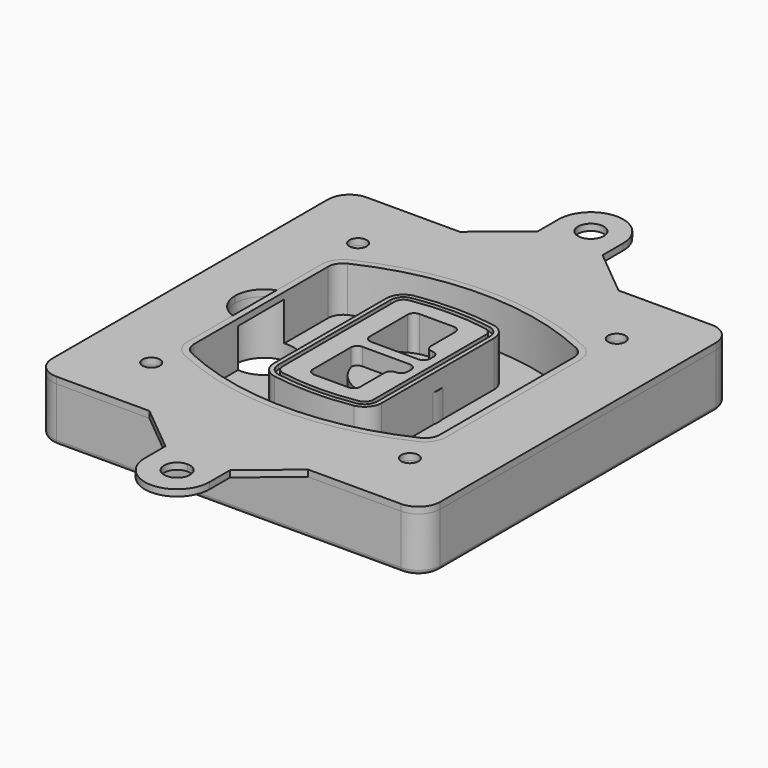
from build123d import *

# Parameters (mm, degrees)
F0_R      = 4
F1_DEPTH  = 25
F2_DEPTH  = 3
F3_DEPTH  = 18
F5_DEPTH  = 21
F6_DEPTH  = 2
F8_DEPTH  = 20
F9_DEPTH  = 16
F10_DEPTH = 25
F7_R      = 6
F7_R_2    = 4
F11_DEPTH = 6
F13_DEPTH = 9
F14_R     = 2
F15_R     = 4
F16_DEPTH = 3


# Not quite as in the source:
# - a feature names something its author has since deleted; it is built from what else it names


with BuildPart() as f1:
    # F0 (on Top) → F1 (new body)
    with BuildSketch(Plane.XY):
        with BuildLine():
            ThreePointArc((-90, -80), (-87.0710678119, -87.0710678119), (-80, -90))
            Line((-80, -90), (80, -90))
            ThreePointArc((80, -90), (87.0710678119, -87.0710678119), (90, -80))
            Line((90, -80), (90, 80))
            ThreePointArc((90, 80), (87.0710678119, 87.0710678119), (80, 90))
            Line((80, 90), (-80, 90))
            ThreePointArc((-80, 90), (-87.0710678119, 87.0710678119), (-90, 80))
            Line((-90, 80), (-90, -80))
        make_face()
        with Locations((-60, -60)):
            Circle(F0_R, mode=Mode.SUBTRACT)
        with Locations((60, -60)):
            Circle(F0_R, mode=Mode.SUBTRACT)
        with BuildLine():
            ThreePointArc((-64, 38.8308515907), (-61.8195654598, 46.3340424013), (-55.9574468085, 51.5000594398))
            ThreePointArc((-55.9574468085, 51.5000594398), (0, 64), (55.9574468085, 51.5000594398))
            ThreePointArc((55.9574468085, 51.5000594398), (61.8195654598, 46.3340424013), (64, 38.8308515907))
            Line((64, 38.8308515907), (64, -38.8308515907))
            ThreePointArc((64, -38.8308515907), (61.8195654598, -46.3340424013), (55.9574468085, -51.5000594398))
            ThreePointArc((55.9574468085, -51.5000594398), (0, -64), (-55.9574468085, -51.5000594398))
            ThreePointArc((-55.9574468085, -51.5000594398), (-61.8195654598, -46.3340424013), (-64, -38.8308515907))
            Line((-64, -38.8308515907), (-64, 38.8308515907))
        make_face(mode=Mode.SUBTRACT)
        with Locations((-60, 60)):
            Circle(F0_R, mode=Mode.SUBTRACT)
        with Locations((60, 60)):
            Circle(F0_R, mode=Mode.SUBTRACT)
        with BuildLine():
            ThreePointArc((55.9574468085, 51.5000594398), (0, 64), (-55.9574468085, 51.5000594398))
            ThreePointArc((-55.9574468085, 51.5000594398), (-61.8195654598, 46.3340424013), (-64, 38.8308515907))
            Line((-64, 38.8308515907), (-64, -38.8308515907))
            ThreePointArc((-64, -38.8308515907), (-61.8195654598, -46.3340424013), (-55.9574468085, -51.5000594398))
            ThreePointArc((-55.9574468085, -51.5000594398), (0, -64), (55.9574468085, -51.5000594398))
            ThreePointArc((55.9574468085, -51.5000594398), (61.8195654598, -46.3340424013), (64, -38.8308515907))
            Line((64, -38.8308515907), (64, 38.8308515907))
            ThreePointArc((64, 38.8308515907), (61.8195654598, 46.3340424013), (55.9574468085, 51.5000594398))
        make_face()
        with BuildLine():
            Line((-60, -38.8308515907), (-60, 38.8308515907))
            ThreePointArc((-60, 38.8308515907), (-58.442546757, 44.1902735983), (-54.2553191489, 47.8802857686))
            ThreePointArc((-54.2553191489, 47.8802857686), (0, 60), (54.2553191489, 47.8802857686))
            ThreePointArc((54.2553191489, 47.8802857686), (58.442546757, 44.1902735983), (60, 38.8308515907))
            Line((60, 38.8308515907), (60, -38.8308515907))
            ThreePointArc((60, -38.8308515907), (58.442546757, -44.1902735983), (54.2553191489, -47.8802857686))
            ThreePointArc((54.2553191489, -47.8802857686), (0, -60), (-54.2553191489, -47.8802857686))
            ThreePointArc((-54.2553191489, -47.8802857686), (-58.442546757, -44.1902735983), (-60, -38.8308515907))
        make_face(mode=Mode.SUBTRACT)
        with BuildLine():
            ThreePointArc((-54.2553191489, 47.8802857686), (-58.442546757, 44.1902735983), (-60, 38.8308515907))
            Line((-60, 38.8308515907), (-60, -38.8308515907))
            ThreePointArc((-60, -38.8308515907), (-58.442546757, -44.1902735983), (-54.2553191489, -47.8802857686))
            ThreePointArc((-54.2553191489, -47.8802857686), (0, -60), (54.2553191489, -47.8802857686))
            ThreePointArc((54.2553191489, -47.8802857686), (58.442546757, -44.1902735983), (60, -38.8308515907))
            Line((60, -38.8308515907), (60, 38.8308515907))
            ThreePointArc((60, 38.8308515907), (58.442546757, 44.1902735983), (54.2553191489, 47.8802857686))
            ThreePointArc((54.2553191489, 47.8802857686), (0, 60), (-54.2553191489, 47.8802857686))
        make_face()
        with BuildLine():
            ThreePointArc((52.9787234043, 45.1654555152), (55.9097827299, 42.582446996), (57, 38.8308515907))
            Line((57, 38.8308515907), (57, -38.8308515907))
            ThreePointArc((57, -38.8308515907), (55.9097827299, -42.582446996), (52.9787234043, -45.1654555152))
            ThreePointArc((52.9787234043, -45.1654555152), (0, -57), (-52.9787234043, -45.1654555152))
            ThreePointArc((-52.9787234043, -45.1654555152), (-55.9097827299, -42.582446996), (-57, -38.8308515907))
            Line((-57, -38.8308515907), (-57, 38.8308515907))
            ThreePointArc((-57, 38.8308515907), (-55.9097827299, 42.582446996), (-52.9787234043, 45.1654555152))
            ThreePointArc((-52.9787234043, 45.1654555152), (0, 57), (52.9787234043, 45.1654555152))
        make_face(mode=Mode.SUBTRACT)
        with BuildLine():
            Line((57, -38.8308515907), (57, 38.8308515907))
            ThreePointArc((57, 38.8308515907), (55.9097827299, 42.582446996), (52.9787234043, 45.1654555152))
            ThreePointArc((52.9787234043, 45.1654555152), (0, 57), (-52.9787234043, 45.1654555152))
            ThreePointArc((-52.9787234043, 45.1654555152), (-55.9097827299, 42.582446996), (-57, 38.8308515907))
            Line((-57, 38.8308515907), (-57, -38.8308515907))
            ThreePointArc((-57, -38.8308515907), (-55.9097827299, -42.582446996), (-52.9787234043, -45.1654555152))
            ThreePointArc((-52.9787234043, -45.1654555152), (0, -57), (52.9787234043, -45.1654555152))
            ThreePointArc((52.9787234043, -45.1654555152), (55.9097827299, -42.582446996), (57, -38.8308515907))
        make_face()
    extrude(amount=-F1_DEPTH)

    # F0 (on Top) → F2 (join)
    with BuildSketch(Plane.XY):
        with BuildLine():
            ThreePointArc((-54.2553191489, 47.8802857686), (-58.442546757, 44.1902735983), (-60, 38.8308515907))
            Line((-60, 38.8308515907), (-60, -38.8308515907))
            ThreePointArc((-60, -38.8308515907), (-58.442546757, -44.1902735983), (-54.2553191489, -47.8802857686))
            ThreePointArc((-54.2553191489, -47.8802857686), (0, -60), (54.2553191489, -47.8802857686))
            ThreePointArc((54.2553191489, -47.8802857686), (58.442546757, -44.1902735983), (60, -38.8308515907))
            Line((60, -38.8308515907), (60, 38.8308515907))
            ThreePointArc((60, 38.8308515907), (58.442546757, 44.1902735983), (54.2553191489, 47.8802857686))
            ThreePointArc((54.2553191489, 47.8802857686), (0, 60), (-54.2553191489, 47.8802857686))
        make_face()
        with BuildLine():
            ThreePointArc((52.9787234043, 45.1654555152), (55.9097827299, 42.582446996), (57, 38.8308515907))
            Line((57, 38.8308515907), (57, -38.8308515907))
            ThreePointArc((57, -38.8308515907), (55.9097827299, -42.582446996), (52.9787234043, -45.1654555152))
            ThreePointArc((52.9787234043, -45.1654555152), (0, -57), (-52.9787234043, -45.1654555152))
            ThreePointArc((-52.9787234043, -45.1654555152), (-55.9097827299, -42.582446996), (-57, -38.8308515907))
            Line((-57, -38.8308515907), (-57, 38.8308515907))
            ThreePointArc((-57, 38.8308515907), (-55.9097827299, 42.582446996), (-52.9787234043, 45.1654555152))
            ThreePointArc((-52.9787234043, 45.1654555152), (0, 57), (52.9787234043, 45.1654555152))
        make_face(mode=Mode.SUBTRACT)
    extrude(amount=F2_DEPTH)

    # F0 (on Top) → F3 (cut)
    with BuildSketch(Plane.XY):
        with BuildLine():
            Line((57, -38.8308515907), (57, 38.8308515907))
            ThreePointArc((57, 38.8308515907), (55.9097827299, 42.582446996), (52.9787234043, 45.1654555152))
            ThreePointArc((52.9787234043, 45.1654555152), (0, 57), (-52.9787234043, 45.1654555152))
            ThreePointArc((-52.9787234043, 45.1654555152), (-55.9097827299, 42.582446996), (-57, 38.8308515907))
            Line((-57, 38.8308515907), (-57, -38.8308515907))
            ThreePointArc((-57, -38.8308515907), (-55.9097827299, -42.582446996), (-52.9787234043, -45.1654555152))
            ThreePointArc((-52.9787234043, -45.1654555152), (0, -57), (52.9787234043, -45.1654555152))
            ThreePointArc((52.9787234043, -45.1654555152), (55.9097827299, -42.582446996), (57, -38.8308515907))
        make_face()
    extrude(amount=-F3_DEPTH, mode=Mode.SUBTRACT)

    # F4 (on face) → F5 (join, through all)
    with BuildSketch(Plane.XY.offset(3)):
        with BuildLine():
            ThreePointArc((-25, -32.5662280692), (-23.1122504785, -37.7276614059), (-18.3399014778, -40.4532214146))
            ThreePointArc((-18.3399014778, -40.4532214146), (0, -42), (18.3399014778, -40.4532214146))
            ThreePointArc((18.3399014778, -40.4532214146), (23.1122504785, -37.7276614059), (25, -32.5662280692))
            Line((25, -32.5662280692), (25, 32.5662280692))
            ThreePointArc((25, 32.5662280692), (23.1122504785, 37.7276614059), (18.3399014778, 40.4532214146))
            ThreePointArc((18.3399014778, 40.4532214146), (0, 42), (-18.3399014778, 40.4532214146))
            ThreePointArc((-18.3399014778, 40.4532214146), (-23.1122504785, 37.7276614059), (-25, 32.5662280692))
            Line((-25, 32.5662280692), (-25, -32.5662280692))
        make_face()
        with BuildLine():
            ThreePointArc((18.0049261084, 38.4814730782), (21.5841878588, 36.4373030717), (23, 32.5662280692))
            Line((23, 32.5662280692), (23, -32.5662280692))
            ThreePointArc((23, -32.5662280692), (21.5841878588, -36.4373030717), (18.0049261084, -38.4814730782))
            ThreePointArc((18.0049261084, -38.4814730782), (0, -40), (-18.0049261084, -38.4814730782))
            ThreePointArc((-18.0049261084, -38.4814730782), (-21.5841878588, -36.4373030717), (-23, -32.5662280692))
            Line((-23, -32.5662280692), (-23, 32.5662280692))
            ThreePointArc((-23, 32.5662280692), (-21.5841878588, 36.4373030717), (-18.0049261084, 38.4814730782))
            ThreePointArc((-18.0049261084, 38.4814730782), (0, 40), (18.0049261084, 38.4814730782))
        make_face(mode=Mode.SUBTRACT)
        with BuildLine():
            Line((23, -32.5662280692), (23, 32.5662280692))
            ThreePointArc((23, 32.5662280692), (21.5841878588, 36.4373030717), (18.0049261084, 38.4814730782))
            ThreePointArc((18.0049261084, 38.4814730782), (0, 40), (-18.0049261084, 38.4814730782))
            ThreePointArc((-18.0049261084, 38.4814730782), (-21.5841878588, 36.4373030717), (-23, 32.5662280692))
            Line((-23, 32.5662280692), (-23, -32.5662280692))
            ThreePointArc((-23, -32.5662280692), (-21.5841878588, -36.4373030717), (-18.0049261084, -38.4814730782))
            ThreePointArc((-18.0049261084, -38.4814730782), (0, -40), (18.0049261084, -38.4814730782))
            ThreePointArc((18.0049261084, -38.4814730782), (21.5841878588, -36.4373030717), (23, -32.5662280692))
        make_face()
        with BuildLine():
            ThreePointArc((17.6699507389, 36.5097247419), (20.0561252392, 35.1469447375), (21, 32.5662280692))
            Line((21, 32.5662280692), (21, -32.5662280692))
            ThreePointArc((21, -32.5662280692), (20.0561252392, -35.1469447375), (17.6699507389, -36.5097247419))
            ThreePointArc((17.6699507389, -36.5097247419), (0, -38), (-17.6699507389, -36.5097247419))
            ThreePointArc((-17.6699507389, -36.5097247419), (-20.0561252392, -35.1469447375), (-21, -32.5662280692))
            Line((-21, -32.5662280692), (-21, 32.5662280692))
            ThreePointArc((-21, 32.5662280692), (-20.0561252392, 35.1469447375), (-17.6699507389, 36.5097247419))
            ThreePointArc((-17.6699507389, 36.5097247419), (0, 38), (17.6699507389, 36.5097247419))
        make_face(mode=Mode.SUBTRACT)
        with BuildLine():
            Line((21, -32.5662280692), (21, 32.5662280692))
            ThreePointArc((21, 32.5662280692), (20.0561252392, 35.1469447375), (17.6699507389, 36.5097247419))
            ThreePointArc((17.6699507389, 36.5097247419), (0, 38), (-17.6699507389, 36.5097247419))
            ThreePointArc((-17.6699507389, 36.5097247419), (-20.0561252392, 35.1469447375), (-21, 32.5662280692))
            Line((-21, 32.5662280692), (-21, -32.5662280692))
            ThreePointArc((-21, -32.5662280692), (-20.0561252392, -35.1469447375), (-17.6699507389, -36.5097247419))
            ThreePointArc((-17.6699507389, -36.5097247419), (0, -38), (17.6699507389, -36.5097247419))
            ThreePointArc((17.6699507389, -36.5097247419), (20.0561252392, -35.1469447375), (21, -32.5662280692))
        make_face()
        with BuildLine():
            Line((-8, -2.5), (14, -2.5))
            ThreePointArc((14, -2.5), (16.1213203436, -3.3786796564), (17, -5.5))
            Line((17, -5.5), (17, -7.5))
            ThreePointArc((17, -7.5), (16.1213203436, -9.6213203436), (14, -10.5))
            ThreePointArc((14, -10.5), (11.8786796564, -11.3786796564), (11, -13.5))
            Line((11, -13.5), (11, -27.5))
            ThreePointArc((11, -27.5), (10.1213203436, -29.6213203436), (8, -30.5))
            Line((8, -30.5), (-8, -30.5))
            ThreePointArc((-8, -30.5), (-10.1213203436, -29.6213203436), (-11, -27.5))
            Line((-11, -27.5), (-11, -5.5))
            ThreePointArc((-11, -5.5), (-10.1213203436, -3.3786796564), (-8, -2.5))
        make_face(mode=Mode.SUBTRACT)
        with BuildLine():
            ThreePointArc((-8, 2.5), (-10.1213203436, 3.3786796564), (-11, 5.5))
            Line((-11, 5.5), (-11, 27.5))
            ThreePointArc((-11, 27.5), (-10.1213203436, 29.6213203436), (-8, 30.5))
            Line((-8, 30.5), (8, 30.5))
            ThreePointArc((8, 30.5), (10.1213203436, 29.6213203436), (11, 27.5))
            Line((11, 27.5), (11, 13.5))
            ThreePointArc((11, 13.5), (11.8786796564, 11.3786796564), (14, 10.5))
            ThreePointArc((14, 10.5), (16.1213203436, 9.6213203436), (17, 7.5))
            Line((17, 7.5), (17, 5.5))
            ThreePointArc((17, 5.5), (16.1213203436, 3.3786796564), (14, 2.5))
            Line((14, 2.5), (-8, 2.5))
        make_face(mode=Mode.SUBTRACT)
    extrude(amount=-F5_DEPTH)

    # F4 (on face) → F6 (cut)
    with BuildSketch(Plane.XY.offset(3)):
        with BuildLine():
            Line((23, -32.5662280692), (23, 32.5662280692))
            ThreePointArc((23, 32.5662280692), (21.5841878588, 36.4373030717), (18.0049261084, 38.4814730782))
            ThreePointArc((18.0049261084, 38.4814730782), (0, 40), (-18.0049261084, 38.4814730782))
            ThreePointArc((-18.0049261084, 38.4814730782), (-21.5841878588, 36.4373030717), (-23, 32.5662280692))
            Line((-23, 32.5662280692), (-23, -32.5662280692))
            ThreePointArc((-23, -32.5662280692), (-21.5841878588, -36.4373030717), (-18.0049261084, -38.4814730782))
            ThreePointArc((-18.0049261084, -38.4814730782), (0, -40), (18.0049261084, -38.4814730782))
            ThreePointArc((18.0049261084, -38.4814730782), (21.5841878588, -36.4373030717), (23, -32.5662280692))
        make_face()
        with BuildLine():
            ThreePointArc((17.6699507389, 36.5097247419), (20.0561252392, 35.1469447375), (21, 32.5662280692))
            Line((21, 32.5662280692), (21, -32.5662280692))
            ThreePointArc((21, -32.5662280692), (20.0561252392, -35.1469447375), (17.6699507389, -36.5097247419))
            ThreePointArc((17.6699507389, -36.5097247419), (0, -38), (-17.6699507389, -36.5097247419))
            ThreePointArc((-17.6699507389, -36.5097247419), (-20.0561252392, -35.1469447375), (-21, -32.5662280692))
            Line((-21, -32.5662280692), (-21, 32.5662280692))
            ThreePointArc((-21, 32.5662280692), (-20.0561252392, 35.1469447375), (-17.6699507389, 36.5097247419))
            ThreePointArc((-17.6699507389, 36.5097247419), (0, 38), (17.6699507389, 36.5097247419))
        make_face(mode=Mode.SUBTRACT)
    extrude(amount=-F6_DEPTH, mode=Mode.SUBTRACT)

    # F7 (on face) → F8 (join)
    with BuildSketch(Plane(origin=(0, 0, -25), x_dir=(1, 0, 0), z_dir=(0, 0, -1))):
        with BuildLine():
            ThreePointArc((-6.71157564, 0), (6.7567035675, 13.4682792075), (20.224982775, 0))
            Line((20.224982775, 0), (25.224982775, 0))
            ThreePointArc((25.224982775, 0), (6.7567035675, 18.4682792075), (-11.71157564, 0))
            Line((-11.71157564, 0), (-6.71157564, 0))
        make_face()
        with BuildLine():
            Line((-6.71157564, 0), (20.224982775, 0))
            ThreePointArc((20.224982775, 0), (6.7567035675, 13.4682792075), (-6.71157564, 0))
        make_face()
        with BuildLine():
            ThreePointArc((-6.71157564, 0), (6.7567035675, -13.4682792075), (20.224982775, 0))
            Line((20.224982775, 0), (-6.71157564, 0))
        make_face()
        with BuildLine():
            Line((25.224982775, 0), (20.224982775, 0))
            ThreePointArc((20.224982775, 0), (6.7567035675, -13.4682792075), (-6.71157564, 0))
            Line((-6.71157564, 0), (-11.71157564, 0))
            ThreePointArc((-11.71157564, 0), (6.7567035675, -18.4682792075), (25.224982775, 0))
        make_face()
    extrude(amount=-F8_DEPTH)

    # F7 (on face) → F9 (cut)
    with BuildSketch(Plane(origin=(0, 0, -25), x_dir=(1, 0, 0), z_dir=(0, 0, -1))):
        with BuildLine():
            Line((-6.71157564, 0), (20.224982775, 0))
            ThreePointArc((20.224982775, 0), (6.7567035675, 13.4682792075), (-6.71157564, 0))
        make_face()
        with BuildLine():
            ThreePointArc((-6.71157564, 0), (6.7567035675, -13.4682792075), (20.224982775, 0))
            Line((20.224982775, 0), (-6.71157564, 0))
        make_face()
    extrude(amount=-F9_DEPTH, mode=Mode.SUBTRACT)

    # F7 (on face) → F10 (cut)
    with BuildSketch(Plane(origin=(0, 0, -25), x_dir=(1, 0, 0), z_dir=(0, 0, -1))):
        with BuildLine():
            Line((-69.0318229325, 0), (-42.0952645175, 0))
            ThreePointArc((-42.0952645175, 0), (-55.563543725, 13.4682792075), (-69.0318229325, 0))
        make_face()
        with BuildLine():
            ThreePointArc((-69.0318229325, 0), (-55.563543725, -13.4682792075), (-42.0952645175, 0))
            Line((-42.0952645175, 0), (-69.0318229325, 0))
        make_face()
    extrude(amount=-F10_DEPTH, mode=Mode.SUBTRACT)

    # F7 (on face) → F11 (cut)
    with BuildSketch(Plane(origin=(0, 0, -25), x_dir=(1, 0, 0), z_dir=(0, 0, -1))):
        with Locations((60, -60)):
            Circle(F7_R)
        with Locations((60, -60)):
            Circle(F7_R_2, mode=Mode.SUBTRACT)
        with Locations((-60, -60)):
            Circle(F7_R)
        with Locations((-60, -60)):
            Circle(F7_R_2, mode=Mode.SUBTRACT)
        with Locations((-60, 60)):
            Circle(F7_R)
        with Locations((-60, 60)):
            Circle(F7_R_2, mode=Mode.SUBTRACT)
        with Locations((60, 60)):
            Circle(F7_R)
        with Locations((60, 60)):
            Circle(F7_R_2, mode=Mode.SUBTRACT)
    extrude(amount=-F11_DEPTH, mode=Mode.SUBTRACT)

    # F12 (on face) → F13 (cut, through all)
    with BuildSketch(Plane(origin=(0, 0, -9), x_dir=(1, 0, 0), z_dir=(0, 0, -1))):
        with BuildLine():
            ThreePointArc((20.224982775, 0), (20.1663399806, 1.2554664788), (19.9909222755, 2.5))
            Line((19.9909222755, 2.5), (14, 2.5))
            ThreePointArc((14, 2.5), (16.1213203436, 3.3786796564), (17, 5.5))
            Line((17, 5.5), (17, 7.5))
            ThreePointArc((17, 7.5), (16.1213203436, 9.6213203436), (14, 10.5))
            ThreePointArc((14, 10.5), (12.1627255951, 11.1284134507), (11.0951631559, 12.750384826))
            ThreePointArc((11.0951631559, 12.750384826), (11.0476113807, 12.7664660322), (11, 12.7823698976))
            Line((11, 12.7823698976), (11, -12.7823698976))
            ThreePointArc((11, -12.7823698976), (11.0476113807, -12.7664660322), (11.0951631559, -12.750384826))
            ThreePointArc((11.0951631559, -12.750384826), (12.1627255951, -11.1284134507), (14, -10.5))
            ThreePointArc((14, -10.5), (16.1213203436, -9.6213203436), (17, -7.5))
            Line((17, -7.5), (17, -5.5))
            ThreePointArc((17, -5.5), (16.1213203436, -3.3786796564), (14, -2.5))
            Line((14, -2.5), (19.9909222755, -2.5))
            ThreePointArc((19.9909222755, -2.5), (20.1663399806, -1.2554664788), (20.224982775, 0))
        make_face()
    extrude(amount=F13_DEPTH, mode=Mode.SUBTRACT)

    # F14
    f14_edges = [f1.edges().sort_by_distance(p)[0] for p in [
        (0, -90, -25),
        (-87.071068, -87.071068, -25),
        (-90, 0, -25),
        (-87.071068, 87.071068, -25),
        (87.071068, -87.071068, -25),
        (0, 90, -25),
        (90, 0, -25),
        (87.071068, 87.071068, -25),
    ]]
    fillet(f14_edges, radius=F14_R)


with BuildPart() as f16:
    # F15 (on face) → F16 (new body, through all)
    with BuildSketch(Plane.XY):
        with BuildLine():
            Line((36.8241705, 90), (0, 90))
            Line((0, 90), (-36.8241705, 90))
            Line((-36.8241705, 90), (-80, 90))
            ThreePointArc((-80, 90), (-87.0710678119, 87.0710678119), (-90, 80))
            Line((-90, 80), (-90, -80))
            ThreePointArc((-90, -80), (-87.0710678119, -87.0710678119), (-80, -90))
            Line((-80, -90), (-36.8241705, -90))
            Line((-36.8241705, -90), (0, -90))
            Line((0, -90), (36.8241705, -90))
            Line((36.8241705, -90), (80, -90))
            ThreePointArc((80, -90), (87.0710678119, -87.0710678119), (90, -80))
            Line((90, -80), (90, 80))
            ThreePointArc((90, 80), (87.0710678119, 87.0710678119), (80, 90))
            Line((80, 90), (36.8241705, 90))
        make_face()
        with Locations((-60, -60)):
            Circle(F15_R, mode=Mode.SUBTRACT)
        with Locations((60, -60)):
            Circle(F15_R, mode=Mode.SUBTRACT)
        with Locations((-60, 60)):
            Circle(F15_R, mode=Mode.SUBTRACT)
        with BuildLine():
            ThreePointArc((-60, 38.8308515907), (-58.442546757, 44.1902735983), (-54.2553191489, 47.8802857686))
            ThreePointArc((-54.2553191489, 47.8802857686), (0, 60), (54.2553191489, 47.8802857686))
            ThreePointArc((54.2553191489, 47.8802857686), (58.442546757, 44.1902735983), (60, 38.8308515907))
            Line((60, 38.8308515907), (60, -38.8308515907))
            ThreePointArc((60, -38.8308515907), (58.442546757, -44.1902735983), (54.2553191489, -47.8802857686))
            ThreePointArc((54.2553191489, -47.8802857686), (0, -60), (-54.2553191489, -47.8802857686))
            ThreePointArc((-54.2553191489, -47.8802857686), (-58.442546757, -44.1902735983), (-60, -38.8308515907))
            Line((-60, -38.8308515907), (-60, -12.7166190685))
            ThreePointArc((-60, -12.7166190685), (-66.5441169481, -7.798817635), (-69.0318229325, 0))
            ThreePointArc((-69.0318229325, 0), (-66.5441169481, 7.798817635), (-60, 12.7166190685))
            Line((-60, 12.7166190685), (-60, 38.8308515907))
        make_face(mode=Mode.SUBTRACT)
        with Locations((60, 60)):
            Circle(F15_R, mode=Mode.SUBTRACT)
        with BuildLine():
            Line((15, -108), (36.8241705, -90))
            Line((36.8241705, -90), (0, -90))
            Line((0, -90), (-36.8241705, -90))
            Line((-36.8241705, -90), (-15, -108))
            Line((-15, -108), (-15, -120))
            ThreePointArc((-15, -120), (0, -135), (15, -120))
            Line((15, -120), (15, -108))
        make_face()
        with BuildLine():
            ThreePointArc((6, -120), (-4.2426406871, -124.2426406871), (0, -114))
            ThreePointArc((0, -114), (4.2426406871, -115.7573593129), (6, -120))
        make_face(mode=Mode.SUBTRACT)
        with BuildLine():
            Line((-36.8241705, 90), (0, 90))
            Line((0, 90), (36.8241705, 90))
            Line((36.8241705, 90), (15, 108))
            Line((15, 108), (15, 120))
            ThreePointArc((15, 120), (0, 135), (-15, 120))
            Line((-15, 120), (-15, 108))
            Line((-15, 108), (-36.8241705, 90))
        make_face()
        with BuildLine():
            ThreePointArc((6, 120), (4.2426406871, 115.7573593129), (0, 114))
            ThreePointArc((0, 114), (-4.2426406871, 124.2426406871), (6, 120))
        make_face(mode=Mode.SUBTRACT)
    extrude(amount=F16_DEPTH)


solid = Compound([f1.part, f16.part])
